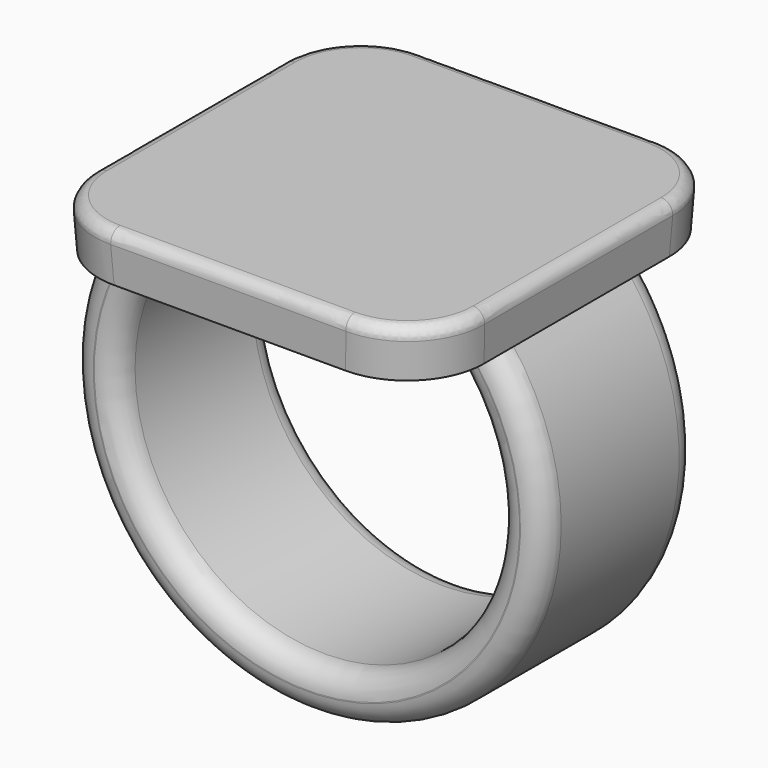
from build123d import *

# Parameters (mm, degrees)
F0_W          = 25.4
F0_H          = 25.4
F1_DEPTH      = 3.175
F1_TAPER      = -3
F3_W          = 4.2106155306
F3_H          = 12.7
F6_DEPTH      = 6.35
F6_DEPTH_BACK = 6.35
F7_R          = 5.08
F8_T4_ANGLE   = 284.1852588065
F8_T9_ANGLE   = 284.1885778804
F8_T14_ANGLE  = 284.1852588065
F8_T19_ANGLE  = 284.1885778804
F8_T24_ANGLE  = 30.6958131666
F8_T29_ANGLE  = 30.6958131666
F9_R          = 0.762


# Not quite as in the source:
# - a fillet or chamfer that OpenCascade refuses, or shapes differently, is made with other operations: its cross-section is extruded or revolved along the edge and cut away or added


with BuildPart() as f1:
    # F0 (on Top) → F1 (new body)
    with BuildSketch(Plane.XY):
        Rectangle(F0_W, F0_H)
    extrude(amount=F1_DEPTH, taper=F1_TAPER)

    # F4: sweep along a path in F2
    with BuildLine(Plane.XZ) as f4_path:
        ThreePointArc((-10.16, 0), (0, -23.5582897328), (10.16, 0))
    # F3 (on face) → F4 (sweep)
    with BuildSketch(Plane(origin=(0, 0, 0), x_dir=(1, 0, 0), z_dir=(0, 0, -1))):
        with Locations((-10.16, 0)):
            Rectangle(F3_W, F3_H)
    sweep(path=f4_path.line)

    # F5 (on Front) → F6 (join, two sides)
    with BuildSketch(Plane.XZ) as f6_sk:
        with BuildLine():
            ThreePointArc((8.0546922347, 0), (9.1072832028, -0.9934796907), (10.0382053359, -2.1017818266))
            Line((10.0382053359, -2.1017818266), (10.16, 0))
            Line((10.16, 0), (8.0546922347, 0))
        make_face()
    extrude(amount=F6_DEPTH)
    extrude(f6_sk.sketch, amount=-F6_DEPTH_BACK)

    # F7
    f7_edges = [f1.edges().sort_by_distance(p)[0] for p in [
        (12.783197, -12.783197, 1.5875),
        (-12.783197, -12.783197, 1.5875),
        (12.783197, 12.783197, 1.5875),
        (-12.783197, 12.783197, 1.5875),
    ]]
    fillet(f7_edges, radius=F7_R)

    # F8: fillet of radius 1.524 on 5 edges, made by hand


with BuildPart() as f8_tool2:
    # F8_s3 → F8_t4 (revolve)
    with BuildSketch(Plane(origin=(-4.6479638678, 0, -3.6193015219), x_dir=(0, 1, 0), z_dir=(0.7890050559, 0, 0.6143867037))):
        with BuildLine():
            ThreePointArc((4.8250343146, 8.0035265624), (5.9036307345, 7.5567572969), (6.3504, 6.478160877))
            Line((6.3504, 6.478160877), (6.5029365685, 6.478160877))
            ThreePointArc((6.5029365685, 6.478160877), (6.5025365685, 7.2406437197), (6.5025365685, 8.0031265624))
            Line((6.5025365685, 8.0031265624), (6.35, 8.1556631309))
            ThreePointArc((6.35, 8.1556631309), (5.5875171573, 8.1556631309), (4.8250343146, 8.1560631309))
            Line((4.8250343146, 8.1560631309), (4.8250343146, 8.0035265624))
        make_face()
    revolve(axis=Axis((0, 6.35, -9.5882897328), (0, -1, 0)), revolution_arc=F8_T4_ANGLE)

    split(bisect_by=Plane.XY, keep=Keep.BOTTOM)


with BuildPart() as f1_1:
    add(f1.part)

    # F8_t1: cut F8_tool2
    add(f8_tool2.part, mode=Mode.SUBTRACT)


with BuildPart() as f8_tool7:
    # F8_s8 → F8_t9 (revolve)
    with BuildSketch(Plane(origin=(-3.393171802, 0, -1.4073750009), x_dir=(0, 1, 0), z_dir=(0.9236987559, 0, 0.3831195746))):
        with BuildLine():
            ThreePointArc((6.3504, 5.1907887924), (5.9036307345, 4.1121923724), (4.8250343146, 3.665423107))
            Line((4.8250343146, 3.665423107), (4.8250343146, 3.5128865384))
            ThreePointArc((4.8250343146, 3.5128865384), (5.5875171573, 3.5132865384), (6.35, 3.5132865384))
            Line((6.35, 3.5132865384), (6.5025365685, 3.665823107))
            ThreePointArc((6.5025365685, 3.665823107), (6.5025365685, 4.4283059497), (6.5029365685, 5.1907887924))
            Line((6.5029365685, 5.1907887924), (6.3504, 5.1907887924))
        make_face()
    revolve(axis=Axis((0, 6.35, -9.5882897328), (0, -1, 0)), revolution_arc=F8_T9_ANGLE)

    split(bisect_by=Plane.XY, keep=Keep.BOTTOM)


with BuildPart() as f1_2:
    add(f1_1.part)

    # F8_t6: cut F8_tool7
    add(f8_tool7.part, mode=Mode.SUBTRACT)


with BuildPart() as f8_tool12:
    # F8_s13 → F8_t14 (revolve)
    with BuildSketch(Plane(origin=(-4.6479638678, 0, -3.6193015219), x_dir=(0, 1, 0), z_dir=(0.7890050559, 0, 0.6143867037))):
        with BuildLine():
            ThreePointArc((-6.3504, 6.478160877), (-5.9036307345, 7.5567572969), (-4.8250343146, 8.0035265624))
            Line((-4.8250343146, 8.0035265624), (-4.8250343146, 8.1560631309))
            ThreePointArc((-4.8250343146, 8.1560631309), (-5.5875171573, 8.1556631309), (-6.35, 8.1556631309))
            Line((-6.35, 8.1556631309), (-6.5025365685, 8.0031265624))
            ThreePointArc((-6.5025365685, 8.0031265624), (-6.5025365685, 7.2406437197), (-6.5029365685, 6.478160877))
            Line((-6.5029365685, 6.478160877), (-6.3504, 6.478160877))
        make_face()
    revolve(axis=Axis((0, -6.35, -9.5882897328), (0, -1, 0)), revolution_arc=F8_T14_ANGLE)

    split(bisect_by=Plane.XY, keep=Keep.BOTTOM)


with BuildPart() as f1_3:
    add(f1_2.part)

    # F8_t11: cut F8_tool12
    add(f8_tool12.part, mode=Mode.SUBTRACT)


with BuildPart() as f8_tool17:
    # F8_s18 → F8_t19 (revolve)
    with BuildSketch(Plane(origin=(-3.393171802, 0, -1.4073750009), x_dir=(0, 1, 0), z_dir=(0.9236987559, 0, 0.3831195746))):
        with BuildLine():
            ThreePointArc((-6.3504, 5.1907887924), (-5.9036307345, 4.1121923724), (-4.8250343146, 3.665423107))
            Line((-4.8250343146, 3.665423107), (-4.8250343146, 3.5128865384))
            ThreePointArc((-4.8250343146, 3.5128865384), (-5.5875171573, 3.5132865384), (-6.35, 3.5132865384))
            Line((-6.35, 3.5132865384), (-6.5025365685, 3.665823107))
            ThreePointArc((-6.5025365685, 3.665823107), (-6.5025365685, 4.4283059497), (-6.5029365685, 5.1907887924))
            Line((-6.5029365685, 5.1907887924), (-6.3504, 5.1907887924))
        make_face()
    revolve(axis=Axis((0, -6.35, -9.5882897328), (0, -1, 0)), revolution_arc=F8_T19_ANGLE)

    split(bisect_by=Plane.XY, keep=Keep.BOTTOM)


with BuildPart() as f1_4:
    add(f1_3.part)

    # F8_t16: cut F8_tool17
    add(f8_tool17.part, mode=Mode.SUBTRACT)


with BuildPart() as f8_tool22:
    # F8_s23 → F8_t24 (revolve)
    with BuildSketch(Plane(origin=(3.4004354425, 0, -1.4146680131), x_dir=(0, 1, 0), z_dir=(-0.9232869408, 0, 0.3841109541))):
        with BuildLine():
            ThreePointArc((-6.3504, -5.1947373949), (-5.9036307345, -4.1161409749), (-4.8250343146, -3.6693717094))
            Line((-4.8250343146, -3.6693717094), (-4.8250343146, -3.5168351409))
            ThreePointArc((-4.8250343146, -3.5168351409), (-5.5875171573, -3.5172351409), (-6.35, -3.5172351409))
            Line((-6.35, -3.5172351409), (-6.5025365685, -3.6697717094))
            ThreePointArc((-6.5025365685, -3.6697717094), (-6.5025365685, -4.4322545521), (-6.5029365685, -5.1947373949))
            Line((-6.5029365685, -5.1947373949), (-6.3504, -5.1947373949))
        make_face()
    revolve(axis=Axis((0, -6.35, -9.5882897328), (0, 1, 0)), revolution_arc=F8_T24_ANGLE)

    split(bisect_by=Plane.XY, keep=Keep.BOTTOM)


with BuildPart() as f1_5:
    add(f1_4.part)

    # F8_t21: cut F8_tool22
    add(f8_tool22.part, mode=Mode.SUBTRACT)


with BuildPart() as f8_tool27:
    # F8_s28 → F8_t29 (revolve)
    with BuildSketch(Plane(origin=(3.4004354425, 0, -1.4146680131), x_dir=(0, 1, 0), z_dir=(-0.9232869408, 0, 0.3841109541))):
        with BuildLine():
            ThreePointArc((6.3504, -5.1947373949), (5.9036307345, -4.1161409749), (4.8250343146, -3.6693717094))
            Line((4.8250343146, -3.6693717094), (4.8250343146, -3.5168351409))
            ThreePointArc((4.8250343146, -3.5168351409), (5.5875171573, -3.5172351409), (6.35, -3.5172351409))
            Line((6.35, -3.5172351409), (6.5025365685, -3.6697717094))
            ThreePointArc((6.5025365685, -3.6697717094), (6.5025365685, -4.4322545521), (6.5029365685, -5.1947373949))
            Line((6.5029365685, -5.1947373949), (6.3504, -5.1947373949))
        make_face()
    revolve(axis=Axis((0, 6.35, -9.5882897328), (0, 1, 0)), revolution_arc=F8_T29_ANGLE)

    split(bisect_by=Plane.XY, keep=Keep.BOTTOM)


with BuildPart() as f1_6:
    add(f1_5.part)

    # F8_t26: cut F8_tool27
    add(f8_tool27.part, mode=Mode.SUBTRACT)

    # F9
    f9_edges = [f1_6.edges().sort_by_distance(p)[0] for p in [
        (-12.866395, 0, 3.175),
        (-11.381378, 11.381378, 3.175),
        (-11.381378, -11.381378, 3.175),
        (0, 12.866395, 3.175),
        (0, -12.866395, 3.175),
        (11.381378, 11.381378, 3.175),
        (11.381378, -11.381378, 3.175),
        (12.866395, 0, 3.175),
    ]]
    fillet(f9_edges, radius=F9_R)


solid = f1_6.part
